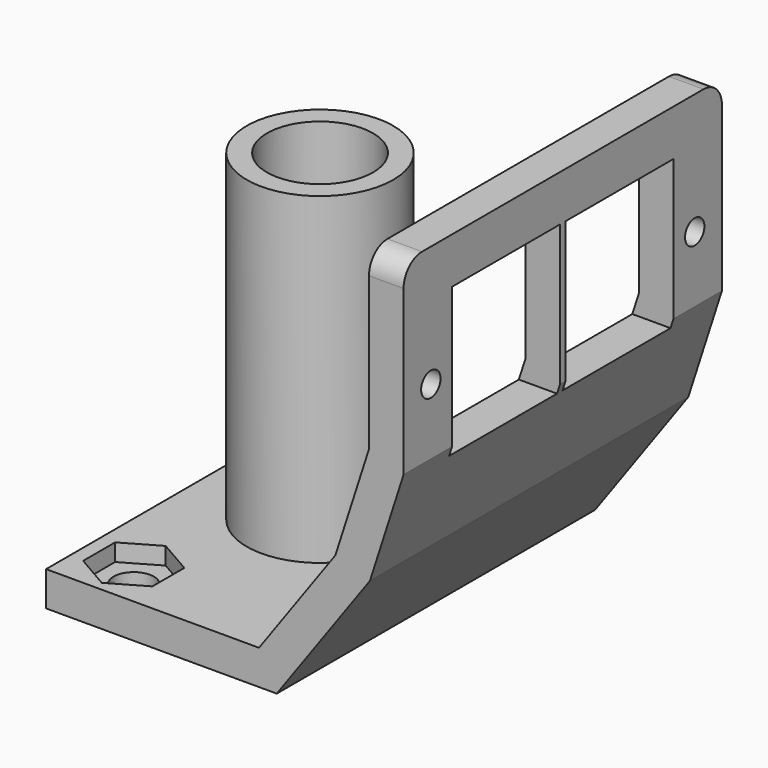
from build123d import *

# Parameters (mm, degrees)
F0_W          = 31
F0_H          = 34.5
F1_DEPTH      = 36.5
F3_DEPTH      = 34.5
F5_R          = 6.35
F5_R_2        = 4.6
F6_DEPTH      = 28
F7_W          = 11.7
F7_H          = 13
F7_R          = 1.05
F8_DEPTH      = 3.0000000261
F4_R          = 1.75
F9_DEPTH      = 3.0000000261
F10_DEPTH     = 1.5
F11_DEPTH     = 3.0000000261
F12_R         = 2
F13_T4_DEPTH  = 47.4768176547
F13_T9_DEPTH  = 47.4768176547
F13_T15_DEPTH = 60.4536353093
F13_T21_DEPTH = 47.4768176547
F13_T23_DEPTH = 60.4536353093


# Not quite as in the source:
# - a fillet or chamfer that OpenCascade refuses, or shapes differently, is made with other operations: its cross-section is extruded or revolved along the edge and cut away or added
# - a feature names something its author has since deleted; it is built from what else it names


with BuildPart() as f1:
    # F0 (on Top) → F1 (new body)
    with BuildSketch(Plane.XY):
        Rectangle(F0_W, F0_H)
    extrude(amount=F1_DEPTH)

    # F2 (on face) → F3 (cut, through all)
    with BuildSketch(Plane.XZ.offset(17.25)):
        Polygon((-15.5, 36.5), (-15.5, 3.0000000261), (2.9619937352, 3.0000000261), (12.4999999739, 16.2664996126), (12.4999999739, 36.5), align=None)
        Polygon((15.5, 15.3), (4.5, 0), (15.5, 0), align=None)
    extrude(amount=-F3_DEPTH, mode=Mode.SUBTRACT)

    # F5 (on face) → F6 (join)
    with BuildSketch(Plane.XY.offset(3.0000000261)):
        with Locations((-5.55, 0)):
            Circle(F5_R)
        with Locations((-5.55, 0)):
            Circle(F5_R_2, mode=Mode.SUBTRACT)
    extrude(amount=F6_DEPTH)

    # F7 (on face) → F8 (cut, through all)
    with BuildSketch(Plane.YZ.offset(15.5)):
        with Locations((6.15, 26)):
            Rectangle(F7_W, F7_H)
        with Locations((-6.15, 26)):
            Rectangle(F7_W, F7_H)
        with Locations((-14.3, 26)):
            Circle(F7_R)
        with Locations((14.3, 26)):
            Circle(F7_R)
    extrude(amount=-F8_DEPTH, mode=Mode.SUBTRACT)

    # F4 (on face) → F9 (cut, through all)
    with BuildSketch(Plane.XY.offset(3.0000000261)):
        with Locations((-11.3, -13)):
            Circle(F4_R)
        with Locations((0.2, 13)):
            Circle(F4_R)
    extrude(amount=-F9_DEPTH, mode=Mode.SUBTRACT)

    # F4 (on face) → F10 (cut)
    with BuildSketch(Plane.XY.offset(3.0000000261)):
        Polygon((-14.3, -11.2679491924), (-14.3, -14.7320508076), (-11.3, -16.4641016151), (-8.3, -14.7320508076), (-8.3, -11.2679491924), (-11.3, -9.5358983849), align=None)
        with Locations((-11.3, -13)):
            Circle(F4_R, mode=Mode.SUBTRACT)
        Polygon((0.2, 16.4641016151), (-2.8, 14.7320508076), (-2.8, 11.2679491924), (0.2, 9.5358983849), (2.9619937352, 11.1305362114), (2.9619937352, 14.8694637886), align=None)
        with Locations((0.2, 13)):
            Circle(F4_R, mode=Mode.SUBTRACT)
    extrude(amount=-F10_DEPTH, mode=Mode.SUBTRACT)

    # F5 (on face) → F11 (cut, through all)
    with BuildSketch(Plane.XY.offset(3.0000000261)):
        with Locations((-5.55, 0)):
            Circle(F5_R_2)
    extrude(amount=-F11_DEPTH, mode=Mode.SUBTRACT)

    # F12
    f12_edges = [f1.edges().sort_by_distance(p)[0] for p in [
        (14, -17.25, 36.5),
        (14, 17.25, 36.5),
    ]]
    fillet(f12_edges, radius=F12_R)

    # F13: chamfer of 5 on 2 edges, made by hand


with BuildPart() as f13_tool2:
    # F13_s3 → F13_t4 (new body)
    with BuildSketch(Plane.XZ.offset(17.25)):
        Polygon((12.4999999739, 21.2664996126), (9.5812730216, 12.2068157607), (12.4999999739, 16.2664996126), align=None)
    extrude(amount=-F13_T4_DEPTH)

    split(bisect_by=Plane.XZ.offset(12), keep=Keep.TOP)


with BuildPart() as f1_1:
    add(f1.part)

    # F13_t1: union F13_tool2
    add(f13_tool2.part)


with BuildPart() as f13_tool7:
    # F13_s8 → F13_t9 (new body)
    with BuildSketch(Plane.XZ.offset(30.2268176547)):
        Polygon((12.4999999739, 21.2664996126), (9.5812730216, 12.2068157607), (12.4999999739, 16.2664996126), align=None)
    extrude(amount=-F13_T9_DEPTH)

    split(bisect_by=Plane.XY.offset(19.5), keep=Keep.BOTTOM)

    split(bisect_by=Plane.XZ.offset(12), keep=Keep.BOTTOM)


with BuildPart() as f1_2:
    add(f1_1.part)

    # F13_t6: union F13_tool7
    add(f13_tool7.part)


with BuildPart() as f13_tool13:
    # F13_s14 → F13_t15 (new body)
    with BuildSketch(Plane.XZ.offset(30.2268176547)):
        Polygon((12.4999999739, 21.2664996126), (9.5812730216, 12.2068157607), (12.4999999739, 16.2664996126), align=None)
    extrude(amount=-F13_T15_DEPTH)

    split(bisect_by=Plane.XZ.offset(-0.3), keep=Keep.TOP)

    split(bisect_by=Plane.XZ.offset(0.3), keep=Keep.BOTTOM)


with BuildPart() as f1_3:
    add(f1_2.part)

    # F13_t12: union F13_tool13
    add(f13_tool13.part)


with BuildPart() as f13_tool19:
    # F13_s20 → F13_t21 (new body)
    with BuildSketch(Plane.XZ.offset(30.2268176547)):
        Polygon((12.4999999739, 21.2664996126), (9.5812730216, 12.2068157607), (12.4999999739, 16.2664996126), align=None)
    extrude(amount=-F13_T21_DEPTH)

    split(bisect_by=Plane.XZ.offset(-12), keep=Keep.BOTTOM)


with BuildPart() as f1_4:
    add(f1_3.part)

    # F13_t18: union F13_tool19
    add(f13_tool19.part)

    # F13_s24 → F13_t23 (cut)
    with BuildSketch(Plane.XZ.offset(-30.2268176547)):
        Polygon((15.5, 20.3), (12.5812730476, 11.2403161481), (15.5, 15.3), align=None)
    extrude(amount=F13_T23_DEPTH, mode=Mode.SUBTRACT)


solid = f1_4.part
